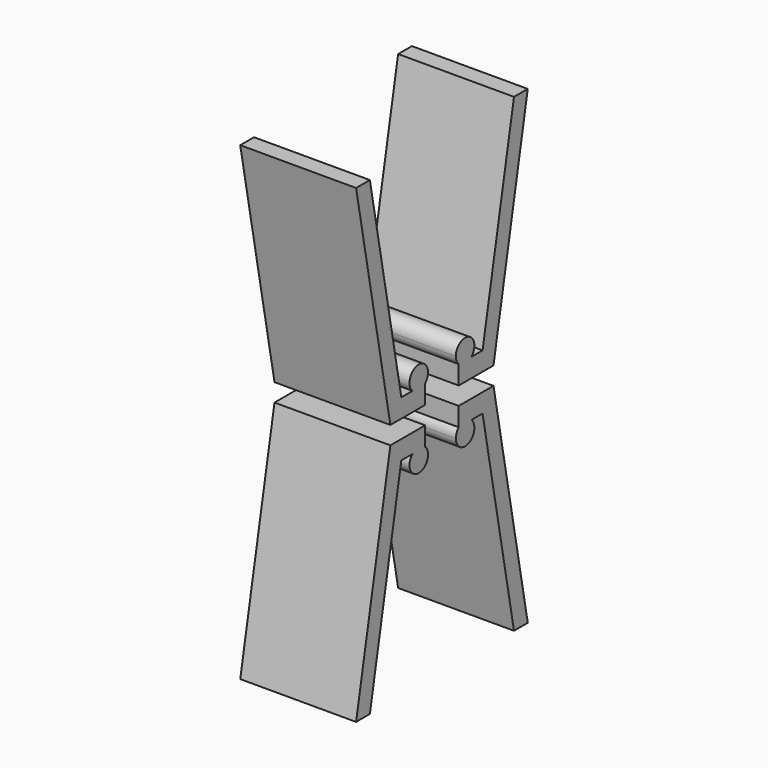
from build123d import *

# Parameters (mm, degrees)
F1_DEPTH = 16
F3_DEPTH = 25
F6_ANGLE = 90


with BuildPart() as f1:
    # F0 (on Front) → F1 (new body)
    with BuildSketch(Plane.XZ):
        with BuildLine():
            ThreePointArc((1.6, 0), (-0.632455532, 1.4696938457), (-1.1, -1.1618950039))
            Line((-1.1, -1.1618950039), (0, -1.1618950039))
            Line((0, -1.1618950039), (1.1, -1.1618950039))
            ThreePointArc((1.1, -1.1618950039), (1.4696938457, -0.632455532), (1.6, 0))
        make_face()
        with BuildLine():
            ThreePointArc((1.1, -1.1618950039), (0, -1.6), (-1.1, -1.1618950039))
            Line((-1.1, -1.1618950039), (-3.0132450199, -1.1618950039))
            Line((-3.0132450199, -1.1618950039), (-4.9, -1.1618950039))
            Line((-4.9, -1.1618950039), (-4.9, -3.7618950039))
            Line((-4.9, -3.7618950039), (1.1, -3.7618950039))
            Line((1.1, -3.7618950039), (1.1, -1.1618950039))
        make_face()
        with BuildLine():
            Line((0, -1.1618950039), (-1.1, -1.1618950039))
            ThreePointArc((-1.1, -1.1618950039), (0, -1.6), (1.1, -1.1618950039))
            Line((1.1, -1.1618950039), (0, -1.1618950039))
        make_face()
        Polygon((-4.9, -1.1618950039), (-3.0132450199, -1.1618950039), (-8.4365460314, 27.4548807241), (-10.8160393536, 27.4548807241), (-4.9, -3.7618950039), align=None)
    extrude(amount=F1_DEPTH)


with BuildPart() as f3:
    # F2 (on face) → F3 (new body)
    with BuildSketch(Plane.XZ.offset(16)):
        with BuildLine():
            Line((4, 0), (1.6, 0))
            ThreePointArc((1.6, 0), (1.4696938457, -0.632455532), (1.1, -1.1618950039))
            Line((1.1, -1.1618950039), (1.1, -3.7618950039))
            Line((1.1, -3.7618950039), (0, -3.7618950039))
            Line((0, -3.7618950039), (0, -5))
            Line((0, -5), (4, -5))
            Line((4, -5), (4, 0))
        make_face()
    extrude(amount=-F3_DEPTH)


with BuildPart() as f4_1:
    # F4: instance of F1
    add(f1.part.mirror(Plane(origin=(4, -3.5, -2.5), x_dir=(0, 1, 0), z_dir=(1, 0, 0))))


with BuildPart() as f5_1:
    # F5: instance of F1
    add(f1.part.mirror(Plane(origin=(2, -3.5, -5), x_dir=(1, 0, 0), z_dir=(0, 0, -1))))


with BuildPart() as f5_2:
    # F5: instance of F4_1
    add(f4_1.part.mirror(Plane(origin=(2, -3.5, -5), x_dir=(1, 0, 0), z_dir=(0, 0, -1))))


with BuildPart() as f5_1_1:
    # F6: moved
    add(f5_1.part.rotate(Axis((4, -16, -2.5), (0, 0, -1)), F6_ANGLE))


with BuildPart() as f4_1_1:
    # F6: moved
    add(f4_1.part.rotate(Axis((4, -16, -2.5), (0, 0, -1)), F6_ANGLE))


with BuildPart() as f5_2_1:
    # F6: moved
    add(f5_2.part.rotate(Axis((4, -16, -2.5), (0, 0, -1)), F6_ANGLE))


with BuildPart() as f1_1:
    # F6: moved
    add(f1.part.rotate(Axis((4, -16, -2.5), (0, 0, -1)), F6_ANGLE))


solid = Compound([f3.part, f5_1_1.part, f4_1_1.part, f5_2_1.part, f1_1.part])
